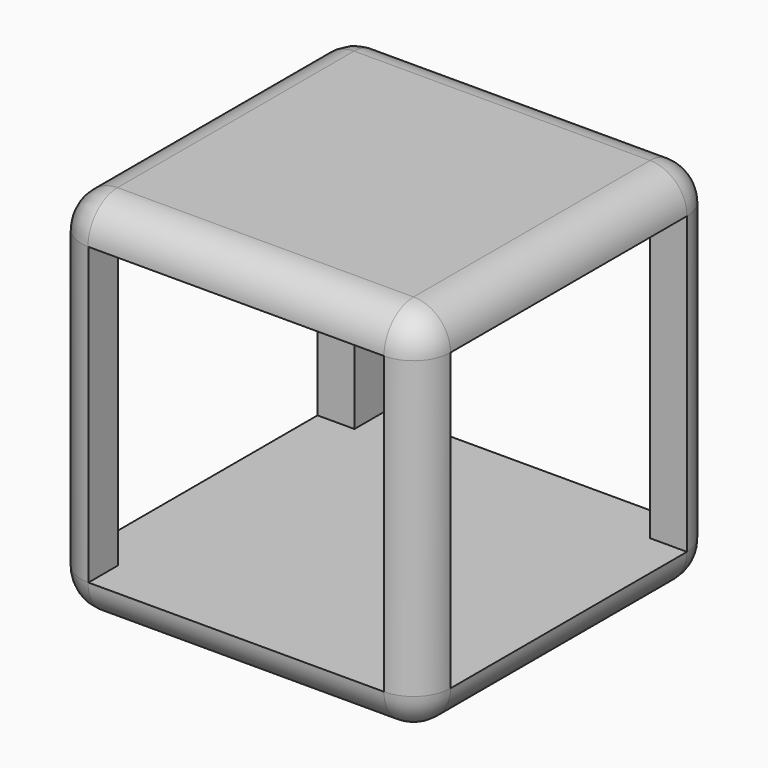
from build123d import *

# Parameters (mm, degrees)
F0_W         = 50.8
F0_H         = 50.8
F1_DEPTH     = 50.8
F2_W         = 40.64
F2_H         = 40.64
F3_DEPTH     = 50.8
F4_W         = 40.64
F4_H         = 40.64
F5_DEPTH     = 50.8
F6_R         = 5.07999
F7_T1_DEPTH  = 58.4224242529
F7_T3_DEPTH  = 58.4224242529
F7_T6_ANGLE  = 90
F7_T8_ANGLE  = 90
F7_T10_ANGLE = 90


# Not quite as in the source:
# - a fillet or chamfer that OpenCascade refuses, or shapes differently, is made with other operations: its cross-section is extruded or revolved along the edge and cut away or added
# - a fillet or chamfer is up to 0.001 mm smaller than in the source, because OpenCascade refuses the exact size


with BuildPart() as f1:
    # F0 (on Front) → F1 (new body)
    with BuildSketch(Plane.XZ):
        with Locations((25.4, 25.4)):
            Rectangle(F0_W, F0_H)
    extrude(amount=F1_DEPTH)

    # F2 (on face) → F3 (cut)
    with BuildSketch(Plane.XZ.offset(50.8)):
        with Locations((25.4, 25.4)):
            Rectangle(F2_W, F2_H)
    extrude(amount=-F3_DEPTH, mode=Mode.SUBTRACT)

    # F4 (on face) → F5 (cut)
    with BuildSketch(Plane.YZ.offset(50.8)):
        with Locations((-25.4, 25.4)):
            Rectangle(F4_W, F4_H)
    extrude(amount=-F5_DEPTH, mode=Mode.SUBTRACT)

    # F6 (radius 5.08 in the source; OpenCascade refuses exactly that, so slightly less here)
    f6_edges = [f1.edges().sort_by_distance(p)[0] for p in [
        (25.4, -50.8, 50.8),
        (50.8, -25.4, 50.8),
        (50.8, -50.8, 25.4),
        (25.4, -50.8, 0),
        (50.8, -25.4, 0),
        (25.4, 0, 0),
        (0, -25.4, 0),
        (50.8, 0, 25.4),
        (25.4, 0, 50.8),
        (0, 0, 25.4),
    ]]
    fillet(f6_edges, radius=F6_R)

    # F7: fillet of radius 5.08 on 3 edges, made by hand

    # F7_s2 → F7_t1 (cut)
    with BuildSketch(Plane.XZ):
        with BuildLine():
            ThreePointArc((-0.0004, 45.7190343146), (1.4878975516, 49.3121024484), (5.0809656854, 50.8004))
            Line((5.0809656854, 50.8004), (5.0809656854, 51.3085365685))
            ThreePointArc((5.0809656854, 51.3085365685), (2.5404828427, 51.3081365685), (0, 51.3081365685))
            Line((0, 51.3081365685), (-0.5081365685, 50.8))
            ThreePointArc((-0.5081365685, 50.8), (-0.5081365685, 48.2595171573), (-0.5085365685, 45.7190343146))
            Line((-0.5085365685, 45.7190343146), (-0.0004, 45.7190343146))
        make_face()
    extrude(amount=F7_T1_DEPTH, mode=Mode.SUBTRACT)

    # F7_s4 → F7_t3 (cut)
    with BuildSketch(Plane.XY):
        with BuildLine():
            ThreePointArc((-0.0004, -45.7190343146), (1.4878975516, -49.3121024484), (5.0809656854, -50.8004))
            Line((5.0809656854, -50.8004), (5.0809656854, -51.3085365685))
            ThreePointArc((5.0809656854, -51.3085365685), (2.5404828427, -51.3081365685), (0, -51.3081365685))
            Line((0, -51.3081365685), (-0.5081365685, -50.8))
            ThreePointArc((-0.5081365685, -50.8), (-0.5081365685, -48.2595171573), (-0.5085365685, -45.7190343146))
            Line((-0.5085365685, -45.7190343146), (-0.0004, -45.7190343146))
        make_face()
    extrude(amount=F7_T3_DEPTH, mode=Mode.SUBTRACT)

    # F7_s5 → F7_t6 (revolve, cut)
    with BuildSketch(Plane.YZ.offset(5.0809656854)):
        with BuildLine():
            ThreePointArc((-45.72041, 0), (-49.3125053774, 1.4878946226), (-50.8004, 5.07999))
            Line((-50.8004, 5.07999), (-50.8004, 0))
            Line((-50.8004, 0), (-45.72041, 0))
        make_face()
    revolve(axis=Axis((5.0809656854, -45.7190343146, 0), (0, 0, -1)), revolution_arc=F7_T6_ANGLE, mode=Mode.SUBTRACT)

    # F7_s7 → F7_t8 (revolve, cut)
    with BuildSketch(Plane.XY.offset(45.7190343146)):
        with BuildLine():
            ThreePointArc((5.07959, 0), (1.4874946226, -1.4878946226), (-0.0004, -5.07999))
            Line((-0.0004, -5.07999), (-0.0004, 0))
            Line((-0.0004, 0), (5.07959, 0))
        make_face()
    revolve(axis=Axis((5.0809656854, 0, 45.7190343146), (0, 1, 0)), revolution_arc=F7_T8_ANGLE, mode=Mode.SUBTRACT)

    # F7_s9 → F7_t10 (revolve, cut)
    with BuildSketch(Plane.XZ.offset(45.72001)):
        with BuildLine():
            ThreePointArc((-0.0003999063, 45.72001), (1.488242525, 49.3124473888), (5.0809656854, 50.8004))
            Line((5.0809656854, 50.8004), (5.0809656854, 51.3085365685))
            ThreePointArc((5.0809656854, 51.3085365685), (2.5404828427, 51.3081365685), (0, 51.3081365685))
            Line((0, 51.3081365685), (-0.5081365685, 50.8))
            Line((-0.5081365685, 50.8), (-0.5085364917, 45.72001))
            Line((-0.5085364917, 45.72001), (-0.0003999063, 45.72001))
        make_face()
    revolve(axis=Axis((0, -45.72001, 45.72001), (1, 0, 0)), revolution_arc=F7_T10_ANGLE, mode=Mode.SUBTRACT)


solid = f1.part
